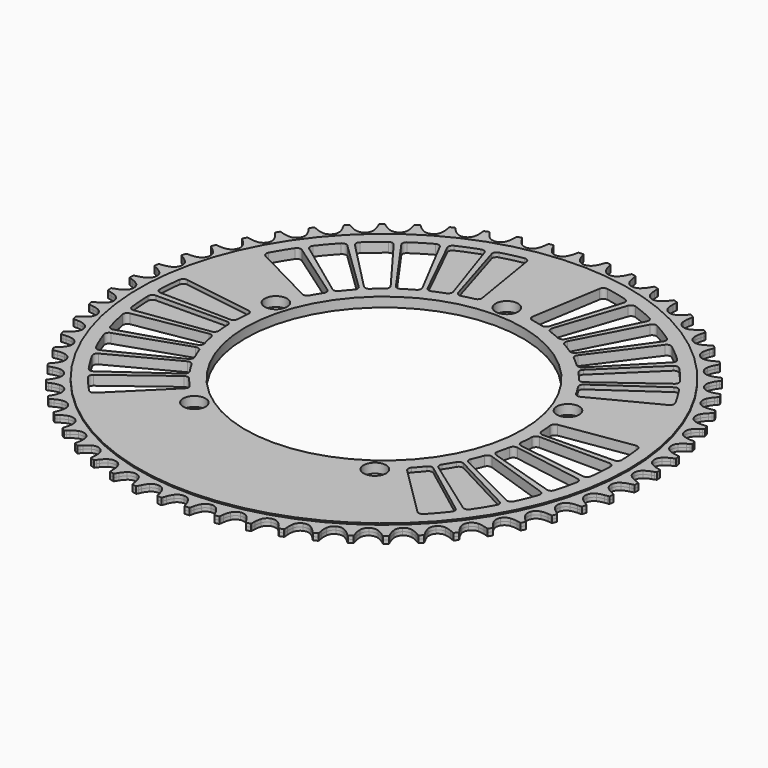
from build123d import *

# Parameters (mm, degrees)
F0_R     = 114.7609592
F0_R_2   = 5.25
F0_R_3   = 64.999997
F1_DEPTH = 2.25
F2_DEPTH = 1.58
F4_DEPTH = 4.5
F5_DEPTH = 2
F6_R     = 2


# Not quite as in the source:
# - the program builds the solid bodies; features that only make, move or delete a surface that nothing else refers to are left out


with BuildPart() as f1:
    # F0 (on Top) → F1 (new body, symmetric)
    with BuildSketch(Plane.XY):
        Circle(F0_R)
        with Locations((-42.3205431025, -58.2492303907)):
            Circle(F0_R_2, mode=Mode.SUBTRACT)
        with Locations((42.3205431025, -58.2492303907)):
            Circle(F0_R_2, mode=Mode.SUBTRACT)
        with Locations((-68.4760771621, 22.2492261907)):
            Circle(F0_R_2, mode=Mode.SUBTRACT)
        Circle(F0_R_3, mode=Mode.SUBTRACT)
        with Locations((68.4760771621, 22.2492261907)):
            Circle(F0_R_2, mode=Mode.SUBTRACT)
        with Locations((0, 72.0000084)):
            Circle(F0_R_2, mode=Mode.SUBTRACT)
    extrude(amount=F1_DEPTH, both=True)

    # F0 (on Top) → F2 (join, symmetric)
    with BuildSketch(Plane.XY):
        with BuildLine():
            ThreePointArc((0, 117.2608808999), (-1.8228579778, 117.698510644), (-3.2483562505, 118.9160021941))
            ThreePointArc((-3.2483562505, 118.9160021941), (-4.0685117692, 120.2255440434), (-4.6854512368, 121.6422093615))
            Line((-4.6854512368, 121.6422093615), (-5.0711986994, 122.7667517072))
            ThreePointArc((-5.0711986994, 122.7667517072), (-5.2354254241, 123.1948132929), (-5.4299253665, 123.6099962774))
            ThreePointArc((-5.4299253665, 123.6099962774), (-6.4754860684, 123.5596347897), (-7.5205832882, 123.5004295385))
            ThreePointArc((-7.5205832882, 123.5004295385), (-7.6706193003, 123.0671901897), (-7.789201754, 122.6243072031))
            Line((-7.789201754, 122.6243072031), (-8.0552893683, 121.4656036285))
            ThreePointArc((-8.0552893683, 121.4656036285), (-8.5207673283, 119.9922112167), (-9.1995455522, 118.6041135787))
            ThreePointArc((-9.1995455522, 118.6041135787), (-10.4899722755, 117.2442864308), (-12.2570996819, 116.6185135251))
            ThreePointArc((-12.2570996819, 116.6185135251), (-14.1157166175, 116.8632053445), (-15.6606683823, 117.9250222046))
            ThreePointArc((-15.6606683823, 117.9250222046), (-16.6132154005, 119.1416606507), (-17.3748570578, 120.4860775935))
            Line((-17.3748570578, 120.4860775935), (-17.8760380386, 121.5641379891))
            ThreePointArc((-17.8760380386, 121.5641379891), (-18.0841097318, 121.9726882415), (-18.3209426226, 122.36526603))
            ThreePointArc((-18.3209426226, 122.36526603), (-19.3555114246, 122.2058895744), (-20.3886948586, 122.0377662494))
            ThreePointArc((-20.3886948586, 122.0377662494), (-20.4926231144, 121.5912171974), (-20.564262083, 121.1383651284))
            Line((-20.564262083, 121.1383651284), (-20.7077745375, 119.9581953238))
            ThreePointArc((-20.7077745375, 119.9581953238), (-21.0166911159, 118.444218614), (-21.5466552087, 116.9927734754))
            ThreePointArc((-21.5466552087, 116.9927734754), (-22.6878721973, 115.5055092806), (-24.3799080147, 114.6984493121))
            ThreePointArc((-24.3799080147, 114.6984493121), (-26.2539205121, 114.7475223121), (-27.9013989542, 115.6420309946))
            ThreePointArc((-27.9013989542, 115.6420309946), (-28.9759011672, 116.7524362919), (-29.8739003088, 118.009875146))
            Line((-29.8739003088, 118.009875146), (-30.4850237643, 119.0296421363))
            ThreePointArc((-30.4850237643, 119.0296421363), (-30.7346607491, 119.4142048932), (-31.0112317974, 119.7798763215))
            ThreePointArc((-31.0112317974, 119.7798763215), (-32.0234737473, 119.5132310597), (-33.0334236215, 119.2380316553))
            ThreePointArc((-33.0334236215, 119.2380316553), (-33.0901054612, 118.7830653848), (-33.1140160532, 118.3252057755))
            Line((-33.1140160532, 118.3252057755), (-33.1333809954, 117.1364999283))
            ThreePointArc((-33.1333809954, 117.1364999283), (-33.2823516376, 115.5985263661), (-33.6576952018, 114.0996360636))
            ThreePointArc((-33.6576952018, 114.0996360636), (-34.6371990436, 112.5012295996), (-36.2356049734, 111.5217248863))
            ThreePointArc((-36.2356049734, 111.5217248863), (-38.1044809596, 111.3746414127), (-39.8364359603, 112.0920414932))
            ThreePointArc((-39.8364359603, 112.0920414932), (-41.0211208971, 113.0840478091), (-42.0456388566, 114.2407318113))
            Line((-42.0456388566, 114.2407318113), (-42.7600091902, 115.1910326156))
            ThreePointArc((-42.7600091902, 115.1910326156), (-43.0484763915, 115.5473945272), (-43.3617554271, 115.8821532224))
            ThreePointArc((-43.3617554271, 115.8821532224), (-44.3405801903, 115.5111605758), (-45.3162312826, 115.1319002342))
            ThreePointArc((-45.3162312826, 115.1319002342), (-45.3250456881, 114.6735014509), (-45.3009659341, 114.2156507071))
            Line((-45.3009659341, 114.2156507071), (-45.1959711976, 113.0314325272))
            ThreePointArc((-45.1959711976, 113.0314325272), (-45.18336375, 111.4863124728), (-45.399974443, 109.9563991622))
            ThreePointArc((-45.399974443, 109.9563991622), (-46.2070334888, 108.2643629048), (-47.6942970613, 107.1231451052))
            ThreePointArc((-47.6942970613, 107.1231451052), (-49.5375607399, 106.7815166354), (-51.3350166378, 107.3139481286))
            ThreePointArc((-51.3350166378, 107.3139481286), (-52.6169046423, 108.1766868341), (-53.7567165864, 109.2199431124))
            Line((-53.7567165864, 109.2199431124), (-54.5665070074, 110.0903660363))
            ThreePointArc((-54.5665070074, 110.0903660363), (-54.8906439181, 110.4146227268), (-55.2371985904, 110.7148010027))
            ThreePointArc((-55.2371985904, 110.7148010027), (-56.1718819578, 110.2435256444), (-57.1025448307, 109.7643596212))
            ThreePointArc((-57.1025448307, 109.7643596212), (-57.0633952296, 109.3075506382), (-56.9915889523, 108.8547250683))
            Line((-56.9915889523, 108.8547250683), (-56.7633848814, 107.6879690979))
            ThreePointArc((-56.7633848814, 107.6879690979), (-56.5893374739, 106.15263121), (-56.6448420636, 104.6084569418))
            ThreePointArc((-56.6448420636, 104.6084569418), (-57.2706140057, 102.8413291941), (-58.6304404499, 101.5509017294))
            ThreePointArc((-58.6304404499, 101.5509017294), (-60.4278966382, 101.0184712164), (-62.2711601305, 101.3601006913))
            ThreePointArc((-62.2711601305, 101.3601006913), (-63.6362065695, 102.0841194408), (-64.87882448, 103.0025178611))
            Line((-64.87882448, 103.0025178611), (-65.7751627549, 103.7835263689))
            ThreePointArc((-65.7751627549, 103.7835263689), (-66.1314180633, 104.0721252141), (-66.5074514467, 104.3344342547))
            ThreePointArc((-66.5074514467, 104.3344342547), (-67.3877528319, 103.768039576), (-68.2632309481, 103.1942177145))
            ThreePointArc((-68.2632309481, 103.1942177145), (-68.1765462717, 102.7440034266), (-68.0578001957, 102.3011642823))
            Line((-68.0578001957, 102.3011642823), (-67.708887042, 101.1646537441))
            ThreePointArc((-67.708887042, 101.1646537441), (-67.3753065744, 99.6559195058), (-67.2690969408, 98.1144025763))
            ThreePointArc((-67.2690969408, 98.1144025763), (-67.706725691, 96.2915443599), (-68.9242164638, 94.8660454234))
            ThreePointArc((-68.9242164638, 94.8660454234), (-70.6561718556, 94.1486462872), (-72.5250477616, 94.2957307799))
            ThreePointArc((-72.5250477616, 94.2957307799), (-73.9582969007, 94.8730970723), (-75.2901063959, 95.6565754694))
            Line((-75.2901063959, 95.6565754694), (-76.263172055, 96.3396126684))
            ThreePointArc((-76.263172055, 96.3396126684), (-76.6476425533, 96.5893917191), (-77.0490347475, 96.8109576116))
            ThreePointArc((-77.0490347475, 96.8109576116), (-77.8653093842, 96.1556491512), (-78.6760108223, 95.4934583638))
            ThreePointArc((-78.6760108223, 95.4934583638), (-78.5427408059, 95.0547714128), (-78.3783559381, 94.6267705326))
            Line((-78.3783559381, 94.6267705326), (-77.9125564672, 93.5329572738))
            ThreePointArc((-77.9125564672, 93.5329572738), (-77.4230977169, 92.0673566932), (-77.156337515, 90.5453862845))
            ThreePointArc((-77.156337515, 90.5453862845), (-77.401028321, 88.6867692154), (-78.4628443387, 87.1418168717))
            ThreePointArc((-78.4628443387, 87.1418168717), (-80.1103232685, 86.2473090875), (-81.9843357927, 86.1982371094))
            ThreePointArc((-81.9843357927, 86.1982371094), (-83.4700846543, 86.6226251989), (-84.8764941506, 87.2625996194))
            Line((-84.8764941506, 87.2625996194), (-85.915626083, 87.8401820112))
            ThreePointArc((-85.915626083, 87.8401820112), (-86.324099432, 88.0484046357), (-86.7464527, 88.2267998579))
            ThreePointArc((-86.7464527, 88.2267998579), (-87.4897573125, 87.4897573125), (-88.2267998579, 86.7464527))
            ThreePointArc((-88.2267998579, 86.7464527), (-88.0484046357, 86.324099432), (-87.8401820112, 85.915626083))
            Line((-87.8401820112, 85.915626083), (-87.2625996194, 84.8764941506))
            ThreePointArc((-87.2625996194, 84.8764941506), (-86.6226251989, 83.4700846543), (-86.1982371094, 81.9843357927))
            ThreePointArc((-86.1982371094, 81.9843357927), (-86.2473090875, 80.1103232685), (-87.1418168717, 78.4628443387))
            ThreePointArc((-87.1418168717, 78.4628443387), (-88.6867692154, 77.401028321), (-90.5453862845, 77.156337515))
            ThreePointArc((-90.5453862845, 77.156337515), (-92.0673566932, 77.4230977169), (-93.5329572738, 77.9125564672))
            Line((-93.5329572738, 77.9125564672), (-94.6267705326, 78.3783559381))
            ThreePointArc((-94.6267705326, 78.3783559381), (-95.0547714128, 78.5427408059), (-95.4934583638, 78.6760108223))
            ThreePointArc((-95.4934583638, 78.6760108223), (-96.1556491512, 77.8653093842), (-96.8109576116, 77.0490347475))
            ThreePointArc((-96.8109576116, 77.0490347475), (-96.5893917191, 76.6476425533), (-96.3396126684, 76.263172055))
            Line((-96.3396126684, 76.263172055), (-95.6565754694, 75.2901063959))
            ThreePointArc((-95.6565754694, 75.2901063959), (-94.8730970723, 73.9582969007), (-94.2957307799, 72.5250477616))
            ThreePointArc((-94.2957307799, 72.5250477616), (-94.1486462872, 70.6561718556), (-94.8660454234, 68.9242164638))
            ThreePointArc((-94.8660454234, 68.9242164638), (-96.2915443599, 67.706725691), (-98.1144025763, 67.2690969408))
            ThreePointArc((-98.1144025763, 67.2690969408), (-99.6559195058, 67.3753065744), (-101.1646537441, 67.708887042))
            Line((-101.1646537441, 67.708887042), (-102.3011642823, 68.0578001957))
            ThreePointArc((-102.3011642823, 68.0578001957), (-102.7440034266, 68.1765462717), (-103.1942177145, 68.2632309481))
            ThreePointArc((-103.1942177145, 68.2632309481), (-103.768039576, 67.3877528319), (-104.3344342547, 66.5074514467))
            ThreePointArc((-104.3344342547, 66.5074514467), (-104.0721252141, 66.1314180633), (-103.7835263689, 65.7751627549))
            Line((-103.7835263689, 65.7751627549), (-103.0025178611, 64.87882448))
            ThreePointArc((-103.0025178611, 64.87882448), (-102.0841194408, 63.6362065695), (-101.3601006913, 62.2711601305))
            ThreePointArc((-101.3601006913, 62.2711601305), (-101.0184712164, 60.4278966382), (-101.5509017294, 58.6304404499))
            ThreePointArc((-101.5509017294, 58.6304404499), (-102.8413291941, 57.2706140057), (-104.6084569418, 56.6448420636))
            ThreePointArc((-104.6084569418, 56.6448420636), (-106.15263121, 56.5893374739), (-107.6879690979, 56.7633848814))
            Line((-107.6879690979, 56.7633848814), (-108.8547250683, 56.9915889523))
            ThreePointArc((-108.8547250683, 56.9915889523), (-109.3075506382, 57.0633952296), (-109.7643596212, 57.1025448307))
            ThreePointArc((-109.7643596212, 57.1025448307), (-110.2435256444, 56.1718819578), (-110.7148010027, 55.2371985904))
            ThreePointArc((-110.7148010027, 55.2371985904), (-110.4146227268, 54.8906439181), (-110.0903660363, 54.5665070074))
            Line((-110.0903660363, 54.5665070074), (-109.2199431124, 53.7567165864))
            ThreePointArc((-109.2199431124, 53.7567165864), (-108.1766868341, 52.6169046423), (-107.3139481286, 51.3350166378))
            ThreePointArc((-107.3139481286, 51.3350166378), (-106.7815166354, 49.5375607399), (-107.1231451052, 47.6942970613))
            ThreePointArc((-107.1231451052, 47.6942970613), (-108.2643629048, 46.2070334888), (-109.9563991622, 45.399974443))
            ThreePointArc((-109.9563991622, 45.399974443), (-111.4863124728, 45.18336375), (-113.0314325272, 45.1959711976))
            Line((-113.0314325272, 45.1959711976), (-114.2156507071, 45.3009659341))
            ThreePointArc((-114.2156507071, 45.3009659341), (-114.6735014509, 45.3250456881), (-115.1319002342, 45.3162312826))
            ThreePointArc((-115.1319002342, 45.3162312826), (-115.5111605758, 44.3405801903), (-115.8821532224, 43.3617554271))
            ThreePointArc((-115.8821532224, 43.3617554271), (-115.5473945272, 43.0484763915), (-115.1910326156, 42.7600091902))
            Line((-115.1910326156, 42.7600091902), (-114.2407318113, 42.0456388566))
            ThreePointArc((-114.2407318113, 42.0456388566), (-113.0840478091, 41.0211208971), (-112.0920414932, 39.8364359603))
            ThreePointArc((-112.0920414932, 39.8364359603), (-111.3746414127, 38.1044809596), (-111.5217248863, 36.2356049734))
            ThreePointArc((-111.5217248863, 36.2356049734), (-112.5012295996, 34.6371990436), (-114.0996360636, 33.6576952018))
            ThreePointArc((-114.0996360636, 33.6576952018), (-115.5985263661, 33.2823516376), (-117.1364999283, 33.1333809954))
            Line((-117.1364999283, 33.1333809954), (-118.3252057755, 33.1140160532))
            ThreePointArc((-118.3252057755, 33.1140160532), (-118.7830653848, 33.0901054612), (-119.2380316553, 33.0334236215))
            ThreePointArc((-119.2380316553, 33.0334236215), (-119.5132310597, 32.0234737473), (-119.7798763215, 31.0112317974))
            ThreePointArc((-119.7798763215, 31.0112317974), (-119.4142048932, 30.7346607491), (-119.0296421363, 30.4850237643))
            Line((-119.0296421363, 30.4850237643), (-118.009875146, 29.8739003088))
            ThreePointArc((-118.009875146, 29.8739003088), (-116.7524362919, 28.9759011672), (-115.6420309946, 27.9013989542))
            ThreePointArc((-115.6420309946, 27.9013989542), (-114.7475223121, 26.2539205121), (-114.6984493121, 24.3799080147))
            ThreePointArc((-114.6984493121, 24.3799080147), (-115.5055092806, 22.6878721973), (-116.9927734754, 21.5466552087))
            ThreePointArc((-116.9927734754, 21.5466552087), (-118.444218614, 21.0166911159), (-119.9581953238, 20.7077745375))
            Line((-119.9581953238, 20.7077745375), (-121.1383651284, 20.564262083))
            ThreePointArc((-121.1383651284, 20.564262083), (-121.5912171974, 20.4926231144), (-122.0377662494, 20.3886948586))
            ThreePointArc((-122.0377662494, 20.3886948586), (-122.2058895744, 19.3555114246), (-122.36526603, 18.3209426226))
            ThreePointArc((-122.36526603, 18.3209426226), (-121.9726882415, 18.0841097318), (-121.5641379891, 17.8760380386))
            Line((-121.5641379891, 17.8760380386), (-120.4860775935, 17.3748570578))
            ThreePointArc((-120.4860775935, 17.3748570578), (-119.1416606507, 16.6132154005), (-117.9250222046, 15.6606683823))
            ThreePointArc((-117.9250222046, 15.6606683823), (-116.8632053445, 14.1157166175), (-116.6185135251, 12.2570996819))
            ThreePointArc((-116.6185135251, 12.2570996819), (-117.2442864308, 10.4899722755), (-118.6041135787, 9.1995455522))
            ThreePointArc((-118.6041135787, 9.1995455522), (-119.9922112167, 8.5207673283), (-121.4656036285, 8.0552893683))
            Line((-121.4656036285, 8.0552893683), (-122.6243072031, 7.789201754))
            ThreePointArc((-122.6243072031, 7.789201754), (-123.0671901897, 7.6706193003), (-123.5004295385, 7.5205832882))
            ThreePointArc((-123.5004295385, 7.5205832882), (-123.5596347897, 6.4754860684), (-123.6099962774, 5.4299253665))
            ThreePointArc((-123.6099962774, 5.4299253665), (-123.1948132929, 5.2354254241), (-122.7667517072, 5.0711986994))
            Line((-122.7667517072, 5.0711986994), (-121.6422093615, 4.6854512368))
            ThreePointArc((-121.6422093615, 4.6854512368), (-120.2255440434, 4.0685117692), (-118.9160021941, 3.2483562505))
            ThreePointArc((-118.9160021941, 3.2483562505), (-117.698510644, 1.8228579778), (-117.2608808999, 0))
            ThreePointArc((-117.2608808999, 0), (-117.698510644, -1.8228579778), (-118.9160021941, -3.2483562505))
            ThreePointArc((-118.9160021941, -3.2483562505), (-120.2255440434, -4.0685117692), (-121.6422093615, -4.6854512368))
            Line((-121.6422093615, -4.6854512368), (-122.7667517072, -5.0711986994))
            ThreePointArc((-122.7667517072, -5.0711986994), (-123.1948132929, -5.2354254241), (-123.6099962774, -5.4299253665))
            ThreePointArc((-123.6099962774, -5.4299253665), (-123.5596347897, -6.4754860684), (-123.5004295385, -7.5205832882))
            ThreePointArc((-123.5004295385, -7.5205832882), (-123.0671901897, -7.6706193003), (-122.6243072031, -7.789201754))
            Line((-122.6243072031, -7.789201754), (-121.4656036285, -8.0552893683))
            ThreePointArc((-121.4656036285, -8.0552893683), (-119.9922112167, -8.5207673283), (-118.6041135787, -9.1995455522))
            ThreePointArc((-118.6041135787, -9.1995455522), (-117.2442864308, -10.4899722755), (-116.6185135251, -12.2570996819))
            ThreePointArc((-116.6185135251, -12.2570996819), (-116.8632053445, -14.1157166175), (-117.9250222046, -15.6606683823))
            ThreePointArc((-117.9250222046, -15.6606683823), (-119.1416606507, -16.6132154005), (-120.4860775935, -17.3748570578))
            Line((-120.4860775935, -17.3748570578), (-121.5641379891, -17.8760380386))
            ThreePointArc((-121.5641379891, -17.8760380386), (-121.9726882415, -18.0841097318), (-122.36526603, -18.3209426226))
            ThreePointArc((-122.36526603, -18.3209426226), (-122.2058895744, -19.3555114246), (-122.0377662494, -20.3886948586))
            ThreePointArc((-122.0377662494, -20.3886948586), (-121.5912171974, -20.4926231144), (-121.1383651284, -20.564262083))
            Line((-121.1383651284, -20.564262083), (-119.9581953238, -20.7077745375))
            ThreePointArc((-119.9581953238, -20.7077745375), (-118.444218614, -21.0166911159), (-116.9927734754, -21.5466552087))
            ThreePointArc((-116.9927734754, -21.5466552087), (-115.5055092806, -22.6878721973), (-114.6984493121, -24.3799080147))
            ThreePointArc((-114.6984493121, -24.3799080147), (-114.7475223121, -26.2539205121), (-115.6420309946, -27.9013989542))
            ThreePointArc((-115.6420309946, -27.9013989542), (-116.7524362919, -28.9759011672), (-118.009875146, -29.8739003088))
            Line((-118.009875146, -29.8739003088), (-119.0296421363, -30.4850237643))
            ThreePointArc((-119.0296421363, -30.4850237643), (-119.4142048932, -30.7346607491), (-119.7798763215, -31.0112317974))
            ThreePointArc((-119.7798763215, -31.0112317974), (-119.5132310597, -32.0234737473), (-119.2380316553, -33.0334236215))
            ThreePointArc((-119.2380316553, -33.0334236215), (-118.7830653848, -33.0901054612), (-118.3252057755, -33.1140160532))
            Line((-118.3252057755, -33.1140160532), (-117.1364999283, -33.1333809954))
            ThreePointArc((-117.1364999283, -33.1333809954), (-115.5985263661, -33.2823516376), (-114.0996360636, -33.6576952018))
            ThreePointArc((-114.0996360636, -33.6576952018), (-112.5012295996, -34.6371990436), (-111.5217248863, -36.2356049734))
            ThreePointArc((-111.5217248863, -36.2356049734), (-111.3746414127, -38.1044809596), (-112.0920414932, -39.8364359603))
            ThreePointArc((-112.0920414932, -39.8364359603), (-113.0840478091, -41.0211208971), (-114.2407318113, -42.0456388566))
            Line((-114.2407318113, -42.0456388566), (-115.1910326156, -42.7600091902))
            ThreePointArc((-115.1910326156, -42.7600091902), (-115.5473945272, -43.0484763915), (-115.8821532224, -43.3617554271))
            ThreePointArc((-115.8821532224, -43.3617554271), (-115.5111605758, -44.3405801903), (-115.1319002342, -45.3162312826))
            ThreePointArc((-115.1319002342, -45.3162312826), (-114.6735014509, -45.3250456881), (-114.2156507071, -45.3009659341))
            Line((-114.2156507071, -45.3009659341), (-113.0314325272, -45.1959711976))
            ThreePointArc((-113.0314325272, -45.1959711976), (-111.4863124728, -45.18336375), (-109.9563991622, -45.399974443))
            ThreePointArc((-109.9563991622, -45.399974443), (-108.2643629048, -46.2070334888), (-107.1231451052, -47.6942970613))
            ThreePointArc((-107.1231451052, -47.6942970613), (-106.7815166354, -49.5375607399), (-107.3139481286, -51.3350166378))
            ThreePointArc((-107.3139481286, -51.3350166378), (-108.1766868341, -52.6169046423), (-109.2199431124, -53.7567165864))
            Line((-109.2199431124, -53.7567165864), (-110.0903660363, -54.5665070074))
            ThreePointArc((-110.0903660363, -54.5665070074), (-110.4146227268, -54.8906439181), (-110.7148010027, -55.2371985904))
            ThreePointArc((-110.7148010027, -55.2371985904), (-110.2435256444, -56.1718819578), (-109.7643596212, -57.1025448307))
            ThreePointArc((-109.7643596212, -57.1025448307), (-109.3075506382, -57.0633952296), (-108.8547250683, -56.9915889523))
            Line((-108.8547250683, -56.9915889523), (-107.6879690979, -56.7633848814))
            ThreePointArc((-107.6879690979, -56.7633848814), (-106.15263121, -56.5893374739), (-104.6084569418, -56.6448420636))
            ThreePointArc((-104.6084569418, -56.6448420636), (-102.8413291941, -57.2706140057), (-101.5509017294, -58.6304404499))
            ThreePointArc((-101.5509017294, -58.6304404499), (-101.0184712164, -60.4278966382), (-101.3601006913, -62.2711601305))
            ThreePointArc((-101.3601006913, -62.2711601305), (-102.0841194408, -63.6362065695), (-103.0025178611, -64.87882448))
            Line((-103.0025178611, -64.87882448), (-103.7835263689, -65.7751627549))
            ThreePointArc((-103.7835263689, -65.7751627549), (-104.0721252141, -66.1314180633), (-104.3344342547, -66.5074514467))
            ThreePointArc((-104.3344342547, -66.5074514467), (-103.768039576, -67.3877528319), (-103.1942177145, -68.2632309481))
            ThreePointArc((-103.1942177145, -68.2632309481), (-102.7440034266, -68.1765462717), (-102.3011642823, -68.0578001957))
            Line((-102.3011642823, -68.0578001957), (-101.1646537441, -67.708887042))
            ThreePointArc((-101.1646537441, -67.708887042), (-99.6559195058, -67.3753065744), (-98.1144025763, -67.2690969408))
            ThreePointArc((-98.1144025763, -67.2690969408), (-96.2915443599, -67.706725691), (-94.8660454234, -68.9242164638))
            ThreePointArc((-94.8660454234, -68.9242164638), (-94.1486462872, -70.6561718556), (-94.2957307799, -72.5250477616))
            ThreePointArc((-94.2957307799, -72.5250477616), (-94.8730970723, -73.9582969007), (-95.6565754694, -75.2901063959))
            Line((-95.6565754694, -75.2901063959), (-96.3396126684, -76.263172055))
            ThreePointArc((-96.3396126684, -76.263172055), (-96.5893917191, -76.6476425533), (-96.8109576116, -77.0490347475))
            ThreePointArc((-96.8109576116, -77.0490347475), (-96.1556491512, -77.8653093842), (-95.4934583638, -78.6760108223))
            ThreePointArc((-95.4934583638, -78.6760108223), (-95.0547714128, -78.5427408059), (-94.6267705326, -78.3783559381))
            Line((-94.6267705326, -78.3783559381), (-93.5329572738, -77.9125564672))
            ThreePointArc((-93.5329572738, -77.9125564672), (-92.0673566932, -77.4230977169), (-90.5453862845, -77.156337515))
            ThreePointArc((-90.5453862845, -77.156337515), (-88.6867692154, -77.401028321), (-87.1418168717, -78.4628443387))
            ThreePointArc((-87.1418168717, -78.4628443387), (-86.2473090875, -80.1103232685), (-86.1982371094, -81.9843357927))
            ThreePointArc((-86.1982371094, -81.9843357927), (-86.6226251989, -83.4700846543), (-87.2625996194, -84.8764941506))
            Line((-87.2625996194, -84.8764941506), (-87.8401820112, -85.915626083))
            ThreePointArc((-87.8401820112, -85.915626083), (-88.0484046357, -86.324099432), (-88.2267998579, -86.7464527))
            ThreePointArc((-88.2267998579, -86.7464527), (-87.4897573125, -87.4897573125), (-86.7464527, -88.2267998579))
            ThreePointArc((-86.7464527, -88.2267998579), (-86.324099432, -88.0484046357), (-85.915626083, -87.8401820112))
            Line((-85.915626083, -87.8401820112), (-84.8764941506, -87.2625996194))
            ThreePointArc((-84.8764941506, -87.2625996194), (-83.4700846543, -86.6226251989), (-81.9843357927, -86.1982371094))
            ThreePointArc((-81.9843357927, -86.1982371094), (-80.1103232685, -86.2473090875), (-78.4628443387, -87.1418168717))
            ThreePointArc((-78.4628443387, -87.1418168717), (-77.401028321, -88.6867692154), (-77.156337515, -90.5453862845))
            ThreePointArc((-77.156337515, -90.5453862845), (-77.4230977169, -92.0673566932), (-77.9125564672, -93.5329572738))
            Line((-77.9125564672, -93.5329572738), (-78.3783559381, -94.6267705326))
            ThreePointArc((-78.3783559381, -94.6267705326), (-78.5427408059, -95.0547714128), (-78.6760108223, -95.4934583638))
            ThreePointArc((-78.6760108223, -95.4934583638), (-77.8653093842, -96.1556491512), (-77.0490347475, -96.8109576116))
            ThreePointArc((-77.0490347475, -96.8109576116), (-76.6476425533, -96.5893917191), (-76.263172055, -96.3396126684))
            Line((-76.263172055, -96.3396126684), (-75.2901063959, -95.6565754694))
            ThreePointArc((-75.2901063959, -95.6565754694), (-73.9582969007, -94.8730970723), (-72.5250477616, -94.2957307799))
            ThreePointArc((-72.5250477616, -94.2957307799), (-70.6561718556, -94.1486462872), (-68.9242164638, -94.8660454234))
            ThreePointArc((-68.9242164638, -94.8660454234), (-67.706725691, -96.2915443599), (-67.2690969408, -98.1144025763))
            ThreePointArc((-67.2690969408, -98.1144025763), (-67.3753065744, -99.6559195058), (-67.708887042, -101.1646537441))
            Line((-67.708887042, -101.1646537441), (-68.0578001957, -102.3011642823))
            ThreePointArc((-68.0578001957, -102.3011642823), (-68.1765462717, -102.7440034266), (-68.2632309481, -103.1942177145))
            ThreePointArc((-68.2632309481, -103.1942177145), (-67.3877528319, -103.768039576), (-66.5074514467, -104.3344342547))
            ThreePointArc((-66.5074514467, -104.3344342547), (-66.1314180633, -104.0721252141), (-65.7751627549, -103.7835263689))
            Line((-65.7751627549, -103.7835263689), (-64.87882448, -103.0025178611))
            ThreePointArc((-64.87882448, -103.0025178611), (-63.6362065695, -102.0841194408), (-62.2711601305, -101.3601006913))
            ThreePointArc((-62.2711601305, -101.3601006913), (-60.4278966382, -101.0184712164), (-58.6304404499, -101.5509017294))
            ThreePointArc((-58.6304404499, -101.5509017294), (-57.2706140057, -102.8413291941), (-56.6448420636, -104.6084569418))
            ThreePointArc((-56.6448420636, -104.6084569418), (-56.5893374739, -106.15263121), (-56.7633848814, -107.6879690979))
            Line((-56.7633848814, -107.6879690979), (-56.9915889523, -108.8547250683))
            ThreePointArc((-56.9915889523, -108.8547250683), (-57.0633952296, -109.3075506382), (-57.1025448307, -109.7643596212))
            ThreePointArc((-57.1025448307, -109.7643596212), (-56.1718819578, -110.2435256444), (-55.2371985904, -110.7148010027))
            ThreePointArc((-55.2371985904, -110.7148010027), (-54.8906439181, -110.4146227268), (-54.5665070074, -110.0903660363))
            Line((-54.5665070074, -110.0903660363), (-53.7567165864, -109.2199431124))
            ThreePointArc((-53.7567165864, -109.2199431124), (-52.6169046423, -108.1766868341), (-51.3350166378, -107.3139481286))
            ThreePointArc((-51.3350166378, -107.3139481286), (-49.5375607399, -106.7815166354), (-47.6942970613, -107.1231451052))
            ThreePointArc((-47.6942970613, -107.1231451052), (-46.2070334888, -108.2643629048), (-45.399974443, -109.9563991622))
            ThreePointArc((-45.399974443, -109.9563991622), (-45.18336375, -111.4863124728), (-45.1959711976, -113.0314325272))
            Line((-45.1959711976, -113.0314325272), (-45.3009659341, -114.2156507071))
            ThreePointArc((-45.3009659341, -114.2156507071), (-45.3250456881, -114.6735014509), (-45.3162312826, -115.1319002342))
            ThreePointArc((-45.3162312826, -115.1319002342), (-44.3405801903, -115.5111605758), (-43.3617554271, -115.8821532224))
            ThreePointArc((-43.3617554271, -115.8821532224), (-43.0484763915, -115.5473945272), (-42.7600091902, -115.1910326156))
            Line((-42.7600091902, -115.1910326156), (-42.0456388566, -114.2407318113))
            ThreePointArc((-42.0456388566, -114.2407318113), (-41.0211208971, -113.0840478091), (-39.8364359603, -112.0920414932))
            ThreePointArc((-39.8364359603, -112.0920414932), (-38.1044809596, -111.3746414127), (-36.2356049734, -111.5217248863))
            ThreePointArc((-36.2356049734, -111.5217248863), (-34.6371990436, -112.5012295996), (-33.6576952018, -114.0996360636))
            ThreePointArc((-33.6576952018, -114.0996360636), (-33.2823516376, -115.5985263661), (-33.1333809954, -117.1364999283))
            Line((-33.1333809954, -117.1364999283), (-33.1140160532, -118.3252057755))
            ThreePointArc((-33.1140160532, -118.3252057755), (-33.0901054612, -118.7830653848), (-33.0334236215, -119.2380316553))
            ThreePointArc((-33.0334236215, -119.2380316553), (-32.0234737473, -119.5132310597), (-31.0112317974, -119.7798763215))
            ThreePointArc((-31.0112317974, -119.7798763215), (-30.7346607491, -119.4142048932), (-30.4850237643, -119.0296421363))
            Line((-30.4850237643, -119.0296421363), (-29.8739003088, -118.009875146))
            ThreePointArc((-29.8739003088, -118.009875146), (-28.9759011672, -116.7524362919), (-27.9013989542, -115.6420309946))
            ThreePointArc((-27.9013989542, -115.6420309946), (-26.2539205121, -114.7475223121), (-24.3799080147, -114.6984493121))
            ThreePointArc((-24.3799080147, -114.6984493121), (-22.6878721973, -115.5055092806), (-21.5466552087, -116.9927734754))
            ThreePointArc((-21.5466552087, -116.9927734754), (-21.0166911159, -118.444218614), (-20.7077745375, -119.9581953238))
            Line((-20.7077745375, -119.9581953238), (-20.564262083, -121.1383651284))
            ThreePointArc((-20.564262083, -121.1383651284), (-20.4926231144, -121.5912171974), (-20.3886948586, -122.0377662494))
            ThreePointArc((-20.3886948586, -122.0377662494), (-19.3555114246, -122.2058895744), (-18.3209426226, -122.36526603))
            ThreePointArc((-18.3209426226, -122.36526603), (-18.0841097318, -121.9726882415), (-17.8760380386, -121.5641379891))
            Line((-17.8760380386, -121.5641379891), (-17.3748570578, -120.4860775935))
            ThreePointArc((-17.3748570578, -120.4860775935), (-16.6132154005, -119.1416606507), (-15.6606683823, -117.9250222046))
            ThreePointArc((-15.6606683823, -117.9250222046), (-14.1157166175, -116.8632053445), (-12.2570996819, -116.6185135251))
            ThreePointArc((-12.2570996819, -116.6185135251), (-10.4899722755, -117.2442864308), (-9.1995455522, -118.6041135787))
            ThreePointArc((-9.1995455522, -118.6041135787), (-8.5207673283, -119.9922112167), (-8.0552893683, -121.4656036285))
            Line((-8.0552893683, -121.4656036285), (-7.789201754, -122.6243072031))
            ThreePointArc((-7.789201754, -122.6243072031), (-7.6706193003, -123.0671901897), (-7.5205832882, -123.5004295385))
            ThreePointArc((-7.5205832882, -123.5004295385), (-6.4754860684, -123.5596347897), (-5.4299253665, -123.6099962774))
            ThreePointArc((-5.4299253665, -123.6099962774), (-5.2354254241, -123.1948132929), (-5.0711986994, -122.7667517072))
            Line((-5.0711986994, -122.7667517072), (-4.6854512368, -121.6422093615))
            ThreePointArc((-4.6854512368, -121.6422093615), (-4.0685117692, -120.2255440434), (-3.2483562505, -118.9160021941))
            ThreePointArc((-3.2483562505, -118.9160021941), (-1.8228579778, -117.698510644), (0, -117.2608808999))
            ThreePointArc((0, -117.2608808999), (1.8228579778, -117.698510644), (3.2483562505, -118.9160021941))
            ThreePointArc((3.2483562505, -118.9160021941), (4.0685117692, -120.2255440434), (4.6854512368, -121.6422093615))
            Line((4.6854512368, -121.6422093615), (5.0711986994, -122.7667517072))
            ThreePointArc((5.0711986994, -122.7667517072), (5.2354254241, -123.1948132929), (5.4299253665, -123.6099962774))
            ThreePointArc((5.4299253665, -123.6099962774), (6.4754860684, -123.5596347897), (7.5205832882, -123.5004295385))
            ThreePointArc((7.5205832882, -123.5004295385), (7.6706193003, -123.0671901897), (7.789201754, -122.6243072031))
            Line((7.789201754, -122.6243072031), (8.0552893683, -121.4656036285))
            ThreePointArc((8.0552893683, -121.4656036285), (8.5207673283, -119.9922112167), (9.1995455522, -118.6041135787))
            ThreePointArc((9.1995455522, -118.6041135787), (10.4899722755, -117.2442864308), (12.2570996819, -116.6185135251))
            ThreePointArc((12.2570996819, -116.6185135251), (14.1157166175, -116.8632053445), (15.6606683823, -117.9250222046))
            ThreePointArc((15.6606683823, -117.9250222046), (16.6132154005, -119.1416606507), (17.3748570578, -120.4860775935))
            Line((17.3748570578, -120.4860775935), (17.8760380386, -121.5641379891))
            ThreePointArc((17.8760380386, -121.5641379891), (18.0841097318, -121.9726882415), (18.3209426226, -122.36526603))
            ThreePointArc((18.3209426226, -122.36526603), (19.3555114246, -122.2058895744), (20.3886948586, -122.0377662494))
            ThreePointArc((20.3886948586, -122.0377662494), (20.4926231144, -121.5912171974), (20.564262083, -121.1383651284))
            Line((20.564262083, -121.1383651284), (20.7077745375, -119.9581953238))
            ThreePointArc((20.7077745375, -119.9581953238), (21.0166911159, -118.444218614), (21.5466552087, -116.9927734754))
            ThreePointArc((21.5466552087, -116.9927734754), (22.6878721973, -115.5055092806), (24.3799080147, -114.6984493121))
            ThreePointArc((24.3799080147, -114.6984493121), (26.2539205121, -114.7475223121), (27.9013989542, -115.6420309946))
            ThreePointArc((27.9013989542, -115.6420309946), (28.9759011672, -116.7524362919), (29.8739003088, -118.009875146))
            Line((29.8739003088, -118.009875146), (30.4850237643, -119.0296421363))
            ThreePointArc((30.4850237643, -119.0296421363), (30.7346607491, -119.4142048932), (31.0112317974, -119.7798763215))
            ThreePointArc((31.0112317974, -119.7798763215), (32.0234737473, -119.5132310597), (33.0334236215, -119.2380316553))
            ThreePointArc((33.0334236215, -119.2380316553), (33.0901054612, -118.7830653848), (33.1140160532, -118.3252057755))
            Line((33.1140160532, -118.3252057755), (33.1333809954, -117.1364999283))
            ThreePointArc((33.1333809954, -117.1364999283), (33.2823516376, -115.5985263661), (33.6576952018, -114.0996360636))
            ThreePointArc((33.6576952018, -114.0996360636), (34.6371990436, -112.5012295996), (36.2356049734, -111.5217248863))
            ThreePointArc((36.2356049734, -111.5217248863), (38.1044809596, -111.3746414127), (39.8364359603, -112.0920414932))
            ThreePointArc((39.8364359603, -112.0920414932), (41.0211208971, -113.0840478091), (42.0456388566, -114.2407318113))
            Line((42.0456388566, -114.2407318113), (42.7600091902, -115.1910326156))
            ThreePointArc((42.7600091902, -115.1910326156), (43.0484763915, -115.5473945272), (43.3617554271, -115.8821532224))
            ThreePointArc((43.3617554271, -115.8821532224), (44.3405801903, -115.5111605758), (45.3162312826, -115.1319002342))
            ThreePointArc((45.3162312826, -115.1319002342), (45.3250456881, -114.6735014509), (45.3009659341, -114.2156507071))
            Line((45.3009659341, -114.2156507071), (45.1959711976, -113.0314325272))
            ThreePointArc((45.1959711976, -113.0314325272), (45.18336375, -111.4863124728), (45.399974443, -109.9563991622))
            ThreePointArc((45.399974443, -109.9563991622), (46.2070334888, -108.2643629048), (47.6942970613, -107.1231451052))
            ThreePointArc((47.6942970613, -107.1231451052), (49.5375607399, -106.7815166354), (51.3350166378, -107.3139481286))
            ThreePointArc((51.3350166378, -107.3139481286), (52.6169046423, -108.1766868341), (53.7567165864, -109.2199431124))
            Line((53.7567165864, -109.2199431124), (54.5665070074, -110.0903660363))
            ThreePointArc((54.5665070074, -110.0903660363), (54.8906439181, -110.4146227268), (55.2371985904, -110.7148010027))
            ThreePointArc((55.2371985904, -110.7148010027), (56.1718819578, -110.2435256444), (57.1025448307, -109.7643596212))
            ThreePointArc((57.1025448307, -109.7643596212), (57.0633952296, -109.3075506382), (56.9915889523, -108.8547250683))
            Line((56.9915889523, -108.8547250683), (56.7633848814, -107.6879690979))
            ThreePointArc((56.7633848814, -107.6879690979), (56.5893374739, -106.15263121), (56.6448420636, -104.6084569418))
            ThreePointArc((56.6448420636, -104.6084569418), (57.2706140057, -102.8413291941), (58.6304404499, -101.5509017294))
            ThreePointArc((58.6304404499, -101.5509017294), (60.4278966382, -101.0184712164), (62.2711601305, -101.3601006913))
            ThreePointArc((62.2711601305, -101.3601006913), (63.6362065695, -102.0841194408), (64.87882448, -103.0025178611))
            Line((64.87882448, -103.0025178611), (65.7751627549, -103.7835263689))
            ThreePointArc((65.7751627549, -103.7835263689), (66.1314180633, -104.0721252141), (66.5074514467, -104.3344342547))
            ThreePointArc((66.5074514467, -104.3344342547), (67.3877528319, -103.768039576), (68.2632309481, -103.1942177145))
            ThreePointArc((68.2632309481, -103.1942177145), (68.1765462717, -102.7440034266), (68.0578001957, -102.3011642823))
            Line((68.0578001957, -102.3011642823), (67.708887042, -101.1646537441))
            ThreePointArc((67.708887042, -101.1646537441), (67.3753065744, -99.6559195058), (67.2690969408, -98.1144025763))
            ThreePointArc((67.2690969408, -98.1144025763), (67.706725691, -96.2915443599), (68.9242164638, -94.8660454234))
            ThreePointArc((68.9242164638, -94.8660454234), (70.6561718556, -94.1486462872), (72.5250477616, -94.2957307799))
            ThreePointArc((72.5250477616, -94.2957307799), (73.9582969007, -94.8730970723), (75.2901063959, -95.6565754694))
            Line((75.2901063959, -95.6565754694), (76.263172055, -96.3396126684))
            ThreePointArc((76.263172055, -96.3396126684), (76.6476425533, -96.5893917191), (77.0490347475, -96.8109576116))
            ThreePointArc((77.0490347475, -96.8109576116), (77.8653093842, -96.1556491512), (78.6760108223, -95.4934583638))
            ThreePointArc((78.6760108223, -95.4934583638), (78.5427408059, -95.0547714128), (78.3783559381, -94.6267705326))
            Line((78.3783559381, -94.6267705326), (77.9125564672, -93.5329572738))
            ThreePointArc((77.9125564672, -93.5329572738), (77.4230977169, -92.0673566932), (77.156337515, -90.5453862845))
            ThreePointArc((77.156337515, -90.5453862845), (77.401028321, -88.6867692154), (78.4628443387, -87.1418168717))
            ThreePointArc((78.4628443387, -87.1418168717), (80.1103232685, -86.2473090875), (81.9843357927, -86.1982371094))
            ThreePointArc((81.9843357927, -86.1982371094), (83.4700846543, -86.6226251989), (84.8764941506, -87.2625996194))
            Line((84.8764941506, -87.2625996194), (85.915626083, -87.8401820112))
            ThreePointArc((85.915626083, -87.8401820112), (86.324099432, -88.0484046357), (86.7464527, -88.2267998579))
            ThreePointArc((86.7464527, -88.2267998579), (87.4897573125, -87.4897573125), (88.2267998579, -86.7464527))
            ThreePointArc((88.2267998579, -86.7464527), (88.0484046357, -86.324099432), (87.8401820112, -85.915626083))
            Line((87.8401820112, -85.915626083), (87.2625996194, -84.8764941506))
            ThreePointArc((87.2625996194, -84.8764941506), (86.6226251989, -83.4700846543), (86.1982371094, -81.9843357927))
            ThreePointArc((86.1982371094, -81.9843357927), (86.2473090875, -80.1103232685), (87.1418168717, -78.4628443387))
            ThreePointArc((87.1418168717, -78.4628443387), (88.6867692154, -77.401028321), (90.5453862845, -77.156337515))
            ThreePointArc((90.5453862845, -77.156337515), (92.0673566932, -77.4230977169), (93.5329572738, -77.9125564672))
            Line((93.5329572738, -77.9125564672), (94.6267705326, -78.3783559381))
            ThreePointArc((94.6267705326, -78.3783559381), (95.0547714128, -78.5427408059), (95.4934583638, -78.6760108223))
            ThreePointArc((95.4934583638, -78.6760108223), (96.1556491512, -77.8653093842), (96.8109576116, -77.0490347475))
            ThreePointArc((96.8109576116, -77.0490347475), (96.5893917191, -76.6476425533), (96.3396126684, -76.263172055))
            Line((96.3396126684, -76.263172055), (95.6565754694, -75.2901063959))
            ThreePointArc((95.6565754694, -75.2901063959), (94.8730970723, -73.9582969007), (94.2957307799, -72.5250477616))
            ThreePointArc((94.2957307799, -72.5250477616), (94.1486462872, -70.6561718556), (94.8660454234, -68.9242164638))
            ThreePointArc((94.8660454234, -68.9242164638), (96.2915443599, -67.706725691), (98.1144025763, -67.2690969408))
            ThreePointArc((98.1144025763, -67.2690969408), (99.6559195058, -67.3753065744), (101.1646537441, -67.708887042))
            Line((101.1646537441, -67.708887042), (102.3011642823, -68.0578001957))
            ThreePointArc((102.3011642823, -68.0578001957), (102.7440034266, -68.1765462717), (103.1942177145, -68.2632309481))
            ThreePointArc((103.1942177145, -68.2632309481), (103.768039576, -67.3877528319), (104.3344342547, -66.5074514467))
            ThreePointArc((104.3344342547, -66.5074514467), (104.0721252141, -66.1314180633), (103.7835263689, -65.7751627549))
            Line((103.7835263689, -65.7751627549), (103.0025178611, -64.87882448))
            ThreePointArc((103.0025178611, -64.87882448), (102.0841194408, -63.6362065695), (101.3601006913, -62.2711601305))
            ThreePointArc((101.3601006913, -62.2711601305), (101.0184712164, -60.4278966382), (101.5509017294, -58.6304404499))
            ThreePointArc((101.5509017294, -58.6304404499), (102.8413291941, -57.2706140057), (104.6084569418, -56.6448420636))
            ThreePointArc((104.6084569418, -56.6448420636), (106.15263121, -56.5893374739), (107.6879690979, -56.7633848814))
            Line((107.6879690979, -56.7633848814), (108.8547250683, -56.9915889523))
            ThreePointArc((108.8547250683, -56.9915889523), (109.3075506382, -57.0633952296), (109.7643596212, -57.1025448307))
            ThreePointArc((109.7643596212, -57.1025448307), (110.2435256444, -56.1718819578), (110.7148010027, -55.2371985904))
            ThreePointArc((110.7148010027, -55.2371985904), (110.4146227268, -54.8906439181), (110.0903660363, -54.5665070074))
            Line((110.0903660363, -54.5665070074), (109.2199431124, -53.7567165864))
            ThreePointArc((109.2199431124, -53.7567165864), (108.1766868341, -52.6169046423), (107.3139481286, -51.3350166378))
            ThreePointArc((107.3139481286, -51.3350166378), (106.7815166354, -49.5375607399), (107.1231451052, -47.6942970613))
            ThreePointArc((107.1231451052, -47.6942970613), (108.2643629048, -46.2070334888), (109.9563991622, -45.399974443))
            ThreePointArc((109.9563991622, -45.399974443), (111.4863124728, -45.18336375), (113.0314325272, -45.1959711976))
            Line((113.0314325272, -45.1959711976), (114.2156507071, -45.3009659341))
            ThreePointArc((114.2156507071, -45.3009659341), (114.6735014509, -45.3250456881), (115.1319002342, -45.3162312826))
            ThreePointArc((115.1319002342, -45.3162312826), (115.5111605758, -44.3405801903), (115.8821532224, -43.3617554271))
            ThreePointArc((115.8821532224, -43.3617554271), (115.5473945272, -43.0484763915), (115.1910326156, -42.7600091902))
            Line((115.1910326156, -42.7600091902), (114.2407318113, -42.0456388566))
            ThreePointArc((114.2407318113, -42.0456388566), (113.0840478091, -41.0211208971), (112.0920414932, -39.8364359603))
            ThreePointArc((112.0920414932, -39.8364359603), (111.3746414127, -38.1044809596), (111.5217248863, -36.2356049734))
            ThreePointArc((111.5217248863, -36.2356049734), (112.5012295996, -34.6371990436), (114.0996360636, -33.6576952018))
            ThreePointArc((114.0996360636, -33.6576952018), (115.5985263661, -33.2823516376), (117.1364999283, -33.1333809954))
            Line((117.1364999283, -33.1333809954), (118.3252057755, -33.1140160532))
            ThreePointArc((118.3252057755, -33.1140160532), (118.7830653848, -33.0901054612), (119.2380316553, -33.0334236215))
            ThreePointArc((119.2380316553, -33.0334236215), (119.5132310597, -32.0234737473), (119.7798763215, -31.0112317974))
            ThreePointArc((119.7798763215, -31.0112317974), (119.4142048932, -30.7346607491), (119.0296421363, -30.4850237643))
            Line((119.0296421363, -30.4850237643), (118.009875146, -29.8739003088))
            ThreePointArc((118.009875146, -29.8739003088), (116.7524362919, -28.9759011672), (115.6420309946, -27.9013989542))
            ThreePointArc((115.6420309946, -27.9013989542), (114.7475223121, -26.2539205121), (114.6984493121, -24.3799080147))
            ThreePointArc((114.6984493121, -24.3799080147), (115.5055092806, -22.6878721973), (116.9927734754, -21.5466552087))
            ThreePointArc((116.9927734754, -21.5466552087), (118.444218614, -21.0166911159), (119.9581953238, -20.7077745375))
            Line((119.9581953238, -20.7077745375), (121.1383651284, -20.564262083))
            ThreePointArc((121.1383651284, -20.564262083), (121.5912171974, -20.4926231144), (122.0377662494, -20.3886948586))
            ThreePointArc((122.0377662494, -20.3886948586), (122.2058895744, -19.3555114246), (122.36526603, -18.3209426226))
            ThreePointArc((122.36526603, -18.3209426226), (121.9726882415, -18.0841097318), (121.5641379891, -17.8760380386))
            Line((121.5641379891, -17.8760380386), (120.4860775935, -17.3748570578))
            ThreePointArc((120.4860775935, -17.3748570578), (119.1416606507, -16.6132154005), (117.9250222046, -15.6606683823))
            ThreePointArc((117.9250222046, -15.6606683823), (116.8632053445, -14.1157166175), (116.6185135251, -12.2570996819))
            ThreePointArc((116.6185135251, -12.2570996819), (117.2442864308, -10.4899722755), (118.6041135787, -9.1995455522))
            ThreePointArc((118.6041135787, -9.1995455522), (119.9922112167, -8.5207673283), (121.4656036285, -8.0552893683))
            Line((121.4656036285, -8.0552893683), (122.6243072031, -7.789201754))
            ThreePointArc((122.6243072031, -7.789201754), (123.0671901897, -7.6706193003), (123.5004295385, -7.5205832882))
            ThreePointArc((123.5004295385, -7.5205832882), (123.5596347897, -6.4754860684), (123.6099962774, -5.4299253665))
            ThreePointArc((123.6099962774, -5.4299253665), (123.1948132929, -5.2354254241), (122.7667517072, -5.0711986994))
            Line((122.7667517072, -5.0711986994), (121.6422093615, -4.6854512368))
            ThreePointArc((121.6422093615, -4.6854512368), (120.2255440434, -4.0685117692), (118.9160021941, -3.2483562505))
            ThreePointArc((118.9160021941, -3.2483562505), (117.698510644, -1.8228579778), (117.2608808999, 0))
            ThreePointArc((117.2608808999, 0), (117.698510644, 1.8228579778), (118.9160021941, 3.2483562505))
            ThreePointArc((118.9160021941, 3.2483562505), (120.2255440434, 4.0685117692), (121.6422093615, 4.6854512368))
            Line((121.6422093615, 4.6854512368), (122.7667517072, 5.0711986994))
            ThreePointArc((122.7667517072, 5.0711986994), (123.1948132929, 5.2354254241), (123.6099962774, 5.4299253665))
            ThreePointArc((123.6099962774, 5.4299253665), (123.5596347897, 6.4754860684), (123.5004295385, 7.5205832882))
            ThreePointArc((123.5004295385, 7.5205832882), (123.0671901897, 7.6706193003), (122.6243072031, 7.789201754))
            Line((122.6243072031, 7.789201754), (121.4656036285, 8.0552893683))
            ThreePointArc((121.4656036285, 8.0552893683), (119.9922112167, 8.5207673283), (118.6041135787, 9.1995455522))
            ThreePointArc((118.6041135787, 9.1995455522), (117.2442864308, 10.4899722755), (116.6185135251, 12.2570996819))
            ThreePointArc((116.6185135251, 12.2570996819), (116.8632053445, 14.1157166175), (117.9250222046, 15.6606683823))
            ThreePointArc((117.9250222046, 15.6606683823), (119.1416606507, 16.6132154005), (120.4860775935, 17.3748570578))
            Line((120.4860775935, 17.3748570578), (121.5641379891, 17.8760380386))
            ThreePointArc((121.5641379891, 17.8760380386), (121.9726882415, 18.0841097318), (122.36526603, 18.3209426226))
            ThreePointArc((122.36526603, 18.3209426226), (122.2058895744, 19.3555114246), (122.0377662494, 20.3886948586))
            ThreePointArc((122.0377662494, 20.3886948586), (121.5912171974, 20.4926231144), (121.1383651284, 20.564262083))
            Line((121.1383651284, 20.564262083), (119.9581953238, 20.7077745375))
            ThreePointArc((119.9581953238, 20.7077745375), (118.444218614, 21.0166911159), (116.9927734754, 21.5466552087))
            ThreePointArc((116.9927734754, 21.5466552087), (115.5055092806, 22.6878721973), (114.6984493121, 24.3799080147))
            ThreePointArc((114.6984493121, 24.3799080147), (114.7475223121, 26.2539205121), (115.6420309946, 27.9013989542))
            ThreePointArc((115.6420309946, 27.9013989542), (116.7524362919, 28.9759011672), (118.009875146, 29.8739003088))
            Line((118.009875146, 29.8739003088), (119.0296421363, 30.4850237643))
            ThreePointArc((119.0296421363, 30.4850237643), (119.4142048932, 30.7346607491), (119.7798763215, 31.0112317974))
            ThreePointArc((119.7798763215, 31.0112317974), (119.5132310597, 32.0234737473), (119.2380316553, 33.0334236215))
            ThreePointArc((119.2380316553, 33.0334236215), (118.7830653848, 33.0901054612), (118.3252057755, 33.1140160532))
            Line((118.3252057755, 33.1140160532), (117.1364999283, 33.1333809954))
            ThreePointArc((117.1364999283, 33.1333809954), (115.5985263661, 33.2823516376), (114.0996360636, 33.6576952018))
            ThreePointArc((114.0996360636, 33.6576952018), (112.5012295996, 34.6371990436), (111.5217248863, 36.2356049734))
            ThreePointArc((111.5217248863, 36.2356049734), (111.3746414127, 38.1044809596), (112.0920414932, 39.8364359603))
            ThreePointArc((112.0920414932, 39.8364359603), (113.0840478091, 41.0211208971), (114.2407318113, 42.0456388566))
            Line((114.2407318113, 42.0456388566), (115.1910326156, 42.7600091902))
            ThreePointArc((115.1910326156, 42.7600091902), (115.5473945272, 43.0484763915), (115.8821532224, 43.3617554271))
            ThreePointArc((115.8821532224, 43.3617554271), (115.5111605758, 44.3405801903), (115.1319002342, 45.3162312826))
            ThreePointArc((115.1319002342, 45.3162312826), (114.6735014509, 45.3250456881), (114.2156507071, 45.3009659341))
            Line((114.2156507071, 45.3009659341), (113.0314325272, 45.1959711976))
            ThreePointArc((113.0314325272, 45.1959711976), (111.4863124728, 45.18336375), (109.9563991622, 45.399974443))
            ThreePointArc((109.9563991622, 45.399974443), (108.2643629048, 46.2070334888), (107.1231451052, 47.6942970613))
            ThreePointArc((107.1231451052, 47.6942970613), (106.7815166354, 49.5375607399), (107.3139481286, 51.3350166378))
            ThreePointArc((107.3139481286, 51.3350166378), (108.1766868341, 52.6169046423), (109.2199431124, 53.7567165864))
            Line((109.2199431124, 53.7567165864), (110.0903660363, 54.5665070074))
            ThreePointArc((110.0903660363, 54.5665070074), (110.4146227268, 54.8906439181), (110.7148010027, 55.2371985904))
            ThreePointArc((110.7148010027, 55.2371985904), (110.2435256444, 56.1718819578), (109.7643596212, 57.1025448307))
            ThreePointArc((109.7643596212, 57.1025448307), (109.3075506382, 57.0633952296), (108.8547250683, 56.9915889523))
            Line((108.8547250683, 56.9915889523), (107.6879690979, 56.7633848814))
            ThreePointArc((107.6879690979, 56.7633848814), (106.15263121, 56.5893374739), (104.6084569418, 56.6448420636))
            ThreePointArc((104.6084569418, 56.6448420636), (102.8413291941, 57.2706140057), (101.5509017294, 58.6304404499))
            ThreePointArc((101.5509017294, 58.6304404499), (101.0184712164, 60.4278966382), (101.3601006913, 62.2711601305))
            ThreePointArc((101.3601006913, 62.2711601305), (102.0841194408, 63.6362065695), (103.0025178611, 64.87882448))
            Line((103.0025178611, 64.87882448), (103.7835263689, 65.7751627549))
            ThreePointArc((103.7835263689, 65.7751627549), (104.0721252141, 66.1314180633), (104.3344342547, 66.5074514467))
            ThreePointArc((104.3344342547, 66.5074514467), (103.768039576, 67.3877528319), (103.1942177145, 68.2632309481))
            ThreePointArc((103.1942177145, 68.2632309481), (102.7440034266, 68.1765462717), (102.3011642823, 68.0578001957))
            Line((102.3011642823, 68.0578001957), (101.1646537441, 67.708887042))
            ThreePointArc((101.1646537441, 67.708887042), (99.6559195058, 67.3753065744), (98.1144025763, 67.2690969408))
            ThreePointArc((98.1144025763, 67.2690969408), (96.2915443599, 67.706725691), (94.8660454234, 68.9242164638))
            ThreePointArc((94.8660454234, 68.9242164638), (94.1486462872, 70.6561718556), (94.2957307799, 72.5250477616))
            ThreePointArc((94.2957307799, 72.5250477616), (94.8730970723, 73.9582969007), (95.6565754694, 75.2901063959))
            Line((95.6565754694, 75.2901063959), (96.3396126684, 76.263172055))
            ThreePointArc((96.3396126684, 76.263172055), (96.5893917191, 76.6476425533), (96.8109576116, 77.0490347475))
            ThreePointArc((96.8109576116, 77.0490347475), (96.1556491512, 77.8653093842), (95.4934583638, 78.6760108223))
            ThreePointArc((95.4934583638, 78.6760108223), (95.0547714128, 78.5427408059), (94.6267705326, 78.3783559381))
            Line((94.6267705326, 78.3783559381), (93.5329572738, 77.9125564672))
            ThreePointArc((93.5329572738, 77.9125564672), (92.0673566932, 77.4230977169), (90.5453862845, 77.156337515))
            ThreePointArc((90.5453862845, 77.156337515), (88.6867692154, 77.401028321), (87.1418168717, 78.4628443387))
            ThreePointArc((87.1418168717, 78.4628443387), (86.2473090875, 80.1103232685), (86.1982371094, 81.9843357927))
            ThreePointArc((86.1982371094, 81.9843357927), (86.6226251989, 83.4700846543), (87.2625996194, 84.8764941506))
            Line((87.2625996194, 84.8764941506), (87.8401820112, 85.915626083))
            ThreePointArc((87.8401820112, 85.915626083), (88.0484046357, 86.324099432), (88.2267998579, 86.7464527))
            ThreePointArc((88.2267998579, 86.7464527), (87.4897573125, 87.4897573125), (86.7464527, 88.2267998579))
            ThreePointArc((86.7464527, 88.2267998579), (86.324099432, 88.0484046357), (85.915626083, 87.8401820112))
            Line((85.915626083, 87.8401820112), (84.8764941506, 87.2625996194))
            ThreePointArc((84.8764941506, 87.2625996194), (83.4700846543, 86.6226251989), (81.9843357927, 86.1982371094))
            ThreePointArc((81.9843357927, 86.1982371094), (80.1103232685, 86.2473090875), (78.4628443387, 87.1418168717))
            ThreePointArc((78.4628443387, 87.1418168717), (77.401028321, 88.6867692154), (77.156337515, 90.5453862845))
            ThreePointArc((77.156337515, 90.5453862845), (77.4230977169, 92.0673566932), (77.9125564672, 93.5329572738))
            Line((77.9125564672, 93.5329572738), (78.3783559381, 94.6267705326))
            ThreePointArc((78.3783559381, 94.6267705326), (78.5427408059, 95.0547714128), (78.6760108223, 95.4934583638))
            ThreePointArc((78.6760108223, 95.4934583638), (77.8653093842, 96.1556491512), (77.0490347475, 96.8109576116))
            ThreePointArc((77.0490347475, 96.8109576116), (76.6476425533, 96.5893917191), (76.263172055, 96.3396126684))
            Line((76.263172055, 96.3396126684), (75.2901063959, 95.6565754694))
            ThreePointArc((75.2901063959, 95.6565754694), (73.9582969007, 94.8730970723), (72.5250477616, 94.2957307799))
            ThreePointArc((72.5250477616, 94.2957307799), (70.6561718556, 94.1486462872), (68.9242164638, 94.8660454234))
            ThreePointArc((68.9242164638, 94.8660454234), (67.706725691, 96.2915443599), (67.2690969408, 98.1144025763))
            ThreePointArc((67.2690969408, 98.1144025763), (67.3753065744, 99.6559195058), (67.708887042, 101.1646537441))
            Line((67.708887042, 101.1646537441), (68.0578001957, 102.3011642823))
            ThreePointArc((68.0578001957, 102.3011642823), (68.1765462717, 102.7440034266), (68.2632309481, 103.1942177145))
            ThreePointArc((68.2632309481, 103.1942177145), (67.3877528319, 103.768039576), (66.5074514467, 104.3344342547))
            ThreePointArc((66.5074514467, 104.3344342547), (66.1314180633, 104.0721252141), (65.7751627549, 103.7835263689))
            Line((65.7751627549, 103.7835263689), (64.87882448, 103.0025178611))
            ThreePointArc((64.87882448, 103.0025178611), (63.6362065695, 102.0841194408), (62.2711601305, 101.3601006913))
            ThreePointArc((62.2711601305, 101.3601006913), (60.4278966382, 101.0184712164), (58.6304404499, 101.5509017294))
            ThreePointArc((58.6304404499, 101.5509017294), (57.2706140057, 102.8413291941), (56.6448420636, 104.6084569418))
            ThreePointArc((56.6448420636, 104.6084569418), (56.5893374739, 106.15263121), (56.7633848814, 107.6879690979))
            Line((56.7633848814, 107.6879690979), (56.9915889523, 108.8547250683))
            ThreePointArc((56.9915889523, 108.8547250683), (57.0633952296, 109.3075506382), (57.1025448307, 109.7643596212))
            ThreePointArc((57.1025448307, 109.7643596212), (56.1718819578, 110.2435256444), (55.2371985904, 110.7148010027))
            ThreePointArc((55.2371985904, 110.7148010027), (54.8906439181, 110.4146227268), (54.5665070074, 110.0903660363))
            Line((54.5665070074, 110.0903660363), (53.7567165864, 109.2199431124))
            ThreePointArc((53.7567165864, 109.2199431124), (52.6169046423, 108.1766868341), (51.3350166378, 107.3139481286))
            ThreePointArc((51.3350166378, 107.3139481286), (49.5375607399, 106.7815166354), (47.6942970613, 107.1231451052))
            ThreePointArc((47.6942970613, 107.1231451052), (46.2070334888, 108.2643629048), (45.399974443, 109.9563991622))
            ThreePointArc((45.399974443, 109.9563991622), (45.18336375, 111.4863124728), (45.1959711976, 113.0314325272))
            Line((45.1959711976, 113.0314325272), (45.3009659341, 114.2156507071))
            ThreePointArc((45.3009659341, 114.2156507071), (45.3250456881, 114.6735014509), (45.3162312826, 115.1319002342))
            ThreePointArc((45.3162312826, 115.1319002342), (44.3405801903, 115.5111605758), (43.3617554271, 115.8821532224))
            ThreePointArc((43.3617554271, 115.8821532224), (43.0484763915, 115.5473945272), (42.7600091902, 115.1910326156))
            Line((42.7600091902, 115.1910326156), (42.0456388566, 114.2407318113))
            ThreePointArc((42.0456388566, 114.2407318113), (41.0211208971, 113.0840478091), (39.8364359603, 112.0920414932))
            ThreePointArc((39.8364359603, 112.0920414932), (38.1044809596, 111.3746414127), (36.2356049734, 111.5217248863))
            ThreePointArc((36.2356049734, 111.5217248863), (34.6371990436, 112.5012295996), (33.6576952018, 114.0996360636))
            ThreePointArc((33.6576952018, 114.0996360636), (33.2823516376, 115.5985263661), (33.1333809954, 117.1364999283))
            Line((33.1333809954, 117.1364999283), (33.1140160532, 118.3252057755))
            ThreePointArc((33.1140160532, 118.3252057755), (33.0901054612, 118.7830653848), (33.0334236215, 119.2380316553))
            ThreePointArc((33.0334236215, 119.2380316553), (32.0234737473, 119.5132310597), (31.0112317974, 119.7798763215))
            ThreePointArc((31.0112317974, 119.7798763215), (30.7346607491, 119.4142048932), (30.4850237643, 119.0296421363))
            Line((30.4850237643, 119.0296421363), (29.8739003088, 118.009875146))
            ThreePointArc((29.8739003088, 118.009875146), (28.9759011672, 116.7524362919), (27.9013989542, 115.6420309946))
            ThreePointArc((27.9013989542, 115.6420309946), (26.2539205121, 114.7475223121), (24.3799080147, 114.6984493121))
            ThreePointArc((24.3799080147, 114.6984493121), (22.6878721973, 115.5055092806), (21.5466552087, 116.9927734754))
            ThreePointArc((21.5466552087, 116.9927734754), (21.0166911159, 118.444218614), (20.7077745375, 119.9581953238))
            Line((20.7077745375, 119.9581953238), (20.564262083, 121.1383651284))
            ThreePointArc((20.564262083, 121.1383651284), (20.4926231144, 121.5912171974), (20.3886948586, 122.0377662494))
            ThreePointArc((20.3886948586, 122.0377662494), (19.3555114246, 122.2058895744), (18.3209426226, 122.36526603))
            ThreePointArc((18.3209426226, 122.36526603), (18.0841097318, 121.9726882415), (17.8760380386, 121.5641379891))
            Line((17.8760380386, 121.5641379891), (17.3748570578, 120.4860775935))
            ThreePointArc((17.3748570578, 120.4860775935), (16.6132154005, 119.1416606507), (15.6606683823, 117.9250222046))
            ThreePointArc((15.6606683823, 117.9250222046), (14.1157166175, 116.8632053445), (12.2570996819, 116.6185135251))
            ThreePointArc((12.2570996819, 116.6185135251), (10.4899722755, 117.2442864308), (9.1995455522, 118.6041135787))
            ThreePointArc((9.1995455522, 118.6041135787), (8.5207673283, 119.9922112167), (8.0552893683, 121.4656036285))
            Line((8.0552893683, 121.4656036285), (7.789201754, 122.6243072031))
            ThreePointArc((7.789201754, 122.6243072031), (7.6706193003, 123.0671901897), (7.5205832882, 123.5004295385))
            ThreePointArc((7.5205832882, 123.5004295385), (6.4754860684, 123.5596347897), (5.4299253665, 123.6099962774))
            ThreePointArc((5.4299253665, 123.6099962774), (5.2354254241, 123.1948132929), (5.0711986994, 122.7667517072))
            Line((5.0711986994, 122.7667517072), (4.6854512368, 121.6422093615))
            ThreePointArc((4.6854512368, 121.6422093615), (4.0685117692, 120.2255440434), (3.2483562505, 118.9160021941))
            ThreePointArc((3.2483562505, 118.9160021941), (1.8228579778, 117.698510644), (0, 117.2608808999))
        make_face()
        Circle(F0_R, mode=Mode.SUBTRACT)
    extrude(amount=F2_DEPTH, both=True)

    # F3 (on face) → F4 (cut)
    with BuildSketch(Plane.XY.offset(2.25)):
        with BuildLine():
            ThreePointArc((-58.0374859821, -41.5026781398), (-60.680093791, -37.5332957441), (-63.0516594686, -33.3962619189))
            Line((-63.0516594686, -33.3962619189), (-95.8022588585, -50.7431105893))
            ThreePointArc((-95.8022588585, -50.7431105893), (-92.1988430109, -57.0290226299), (-88.1835990109, -63.0602009206))
            Line((-88.1835990109, -63.0602009206), (-58.0374859821, -41.5026781398))
        make_face()
        with BuildLine():
            ThreePointArc((-63.9042654616, -31.7343178233), (-65.8812798782, -27.3948723944), (-67.5640198238, -22.9330612251))
            Line((-67.5640198238, -22.9330612251), (-102.6584513592, -34.8450633404))
            ThreePointArc((-102.6584513592, -34.8450633404), (-100.1016544531, -41.6244501515), (-97.0977296, -48.2179114147))
            Line((-97.0977296, -48.2179114147), (-63.9042654616, -31.7343178233))
        make_face()
        with BuildLine():
            ThreePointArc((-50.6904769785, -50.2125244894), (-53.9312792213, -46.7144430927), (-56.9311845249, -43.007700479))
            Line((-56.9311845249, -43.007700479), (-86.5026570742, -65.3469692776))
            ThreePointArc((-86.5026570742, -65.3469692776), (-81.9445263783, -70.9790861543), (-77.0203708844, -76.2941579906))
            Line((-77.0203708844, -76.2941579906), (-50.6904769785, -50.2125244894))
        make_face()
        with BuildLine():
            Line((-103.5354102937, -32.1458378329), (-68.1411848799, -21.1565827834))
            ThreePointArc((-68.1411848799, -21.1565827834), (-69.4021827155, -16.5577506389), (-70.3531791267, -11.8849593467))
            Line((-70.3531791267, -11.8849593467), (-106.8963693424, -18.0583026909))
            ThreePointArc((-106.8963693424, -18.0583026909), (-105.4514017536, -25.1582579458), (-103.5354102937, -32.1458378329))
        make_face()
        with BuildLine():
            ThreePointArc((-63.4191674546, 32.6929850468), (-61.0937573161, 36.8561377371), (-58.4954573195, 40.8546636858))
            Line((-58.4954573195, 40.8546636858), (-88.8794520461, 62.0755916496))
            ThreePointArc((-88.8794520461, 62.0755916496), (-92.8273736546, 56.0001319199), (-96.3606596285, 49.6745342265))
            Line((-96.3606596285, 49.6745342265), (-63.4191674546, 32.6929850468))
        make_face()
        with BuildLine():
            ThreePointArc((-49.9286337968, 50.970124574), (-46.4125069973, 54.1913394015), (-42.6890676505, 57.1704956689))
            Line((-42.6890676505, 57.1704956689), (-64.8628306368, 86.8662723757))
            ThreePointArc((-64.8628306368, 86.8662723757), (-70.5203169448, 82.3396682812), (-75.8628074147, 77.4452743931))
            Line((-75.8628074147, 77.4452743931), (-49.9286337968, 50.970124574))
        make_face()
        with BuildLine():
            Line((-62.5667098431, 88.5344164383), (-41.1778900634, 58.2683742851))
            ThreePointArc((-41.1778900634, 58.2683742851), (-37.1938105461, 60.8887717807), (-33.043595991, 63.2371950349))
            Line((-33.043595991, 63.2371950349), (-50.2072612112, 96.0841662103))
            ThreePointArc((-50.2072612112, 96.0841662103), (-56.5132003805, 92.5159135361), (-62.5667098431, 88.5344164383))
        make_face()
        with BuildLine():
            ThreePointArc((-57.4059619678, 42.3718963754), (-54.4474656972, 46.1117723695), (-51.2457668172, 49.6456791193))
            Line((-51.2457668172, 49.6456791193), (-77.8640920698, 75.4328790436))
            ThreePointArc((-77.8640920698, 75.4328790436), (-82.7288329422, 70.0633732751), (-87.2240457239, 64.3809127165))
            Line((-87.2240457239, 64.3809127165), (-57.4059619678, 42.3718963754))
        make_face()
        with BuildLine():
            ThreePointArc((11.4952759533, 70.417900442), (16.1732606994, 69.4927889083), (20.7790037139, 68.2572712358))
            Line((20.7790037139, 68.2572712358), (31.5721348082, 103.7117947888))
            ThreePointArc((31.5721348082, 103.7117947888), (24.5740543734, 105.5890710553), (17.4662080556, 106.9947085179))
            Line((17.4662080556, 106.9947085179), (11.4952759533, 70.417900442))
        make_face()
        with BuildLine():
            ThreePointArc((22.5586503291, 67.6899502676), (27.0297093889, 66.03193835), (31.3800337961, 64.0789790092))
            Line((31.3800337961, 64.0789790092), (47.6796034562, 97.3631937075))
            ThreePointArc((47.6796034562, 97.3631937075), (41.069612403, 100.3305686804), (34.2761741172, 102.8497932062))
            Line((34.2761741172, 102.8497932062), (22.5586503291, 67.6899502676))
        make_face()
        with BuildLine():
            ThreePointArc((33.0466727634, 63.2355872209), (37.1967730508, 60.8869620404), (41.1807250677, 58.2663707021))
            Line((41.1807250677, 58.2663707021), (62.5710174191, 88.5313721446))
            ThreePointArc((62.5710174191, 88.5313721446), (56.5177016838, 92.5131637717), (50.2119361357, 96.0817232577))
            Line((50.2119361357, 96.0817232577), (33.0466727634, 63.2355872209))
        make_face()
        with BuildLine():
            Line((64.8670570464, 86.8631163659), (42.6918492357, 57.1684185608))
            ThreePointArc((42.6918492357, 57.1684185608), (46.4151436269, 54.1890811326), (49.9311136937, 50.9676952314))
            Line((49.9311136937, 50.9676952314), (75.8665754318, 77.4415831896))
            ThreePointArc((75.8665754318, 77.4415831896), (70.5243231054, 82.3362370113), (64.8670570464, 86.8631163659))
        make_face()
        with BuildLine():
            Line((107.1553698615, 16.451832254), (70.5236387038, 10.8276708428))
            ThreePointArc((70.5236387038, 10.8276708428), (71.0893821373, 6.0927677812), (71.3375878671, 1.3306499172))
            Line((71.3375878671, 1.3306499172), (108.392104455, 2.0218225642))
            ThreePointArc((108.392104455, 2.0218225642), (108.0149744987, 9.2575028328), (107.1553698615, 16.451832254))
        make_face()
        with BuildLine():
            Line((108.4078863327, -0.8162447792), (71.3479746115, -0.5372064133))
            ThreePointArc((71.3479746115, -0.5372064133), (71.1527448055, -5.3017901262), (70.6396942713, -10.0426921273))
            Line((70.6396942713, -10.0426921273), (107.3317075758, -15.2591160791))
            ThreePointArc((107.3317075758, -15.2591160791), (108.111249312, -8.05567172), (108.4078863327, -0.8162447792))
        make_face()
        with BuildLine():
            Line((106.8954905875, -18.0635037222), (70.3526007796, -11.8883823729))
            ThreePointArc((70.3526007796, -11.8883823729), (69.4013770145, -16.5611273888), (68.1401554237, -21.1598981739))
            Line((68.1401554237, -21.1598981739), (103.5338461125, -32.1508753197))
            ThreePointArc((103.5338461125, -32.1508753197), (105.4501775514, -25.1633886636), (106.8954905875, -18.0635037222))
        make_face()
        with BuildLine():
            Line((102.6567558479, -34.8500581555), (67.5629039336, -22.9363485315))
            ThreePointArc((67.5629039336, -22.9363485315), (65.8799469003, -27.3980778216), (63.9027213498, -31.7374270536))
            Line((63.9027213498, -31.7374270536), (97.0953834382, -48.2226356565))
            ThreePointArc((97.0953834382, -48.2226356565), (100.0996290932, -41.6293205573), (102.6567558479, -34.8500581555))
        make_face()
    extrude(amount=-F4_DEPTH, mode=Mode.SUBTRACT)

    # F3 (on face) → F5 (cut)
    with BuildSketch(Plane.XY.offset(2.25)):
        with BuildLine():
            ThreePointArc((-70.6401828157, -10.0392551346), (-71.1530026804, -5.2983281766), (-71.3480006649, -0.5337349704))
            Line((-71.3480006649, -0.5337349704), (-108.4079259189, -0.8109701827))
            ThreePointArc((-108.4079259189, -0.8109701827), (-108.1116411335, -8.0504115478), (-107.3324498825, -15.2538938271))
            Line((-107.3324498825, -15.2538938271), (-70.6401828157, -10.0392551346))
        make_face()
        with BuildLine():
            ThreePointArc((-71.3375230398, 1.3341208525), (-71.0892338942, 6.0944972096), (-70.5236387038, 10.8276708428))
            Line((-70.5236387038, 10.8276708428), (-107.1553698615, 16.451832254))
            ThreePointArc((-107.1553698615, 16.451832254), (-108.0147492545, 9.2601305692), (-108.3920059547, 2.0270963895))
            Line((-108.3920059547, 2.0270963895), (-71.3375230398, 1.3341208525))
        make_face()
        with BuildLine():
            ThreePointArc((-31.3769159904, 64.0805057317), (-27.0264965669, 66.0332534048), (-22.5553568417, 67.6910477807))
            Line((-22.5553568417, 67.6910477807), (-34.2711699106, 102.8514607948))
            ThreePointArc((-34.2711699106, 102.8514607948), (-41.0647307614, 100.3325668074), (-47.6748661847, 97.3655134477))
            Line((-47.6748661847, 97.3655134477), (-31.3769159904, 64.0805057317))
        make_face()
        with BuildLine():
            ThreePointArc((-20.7756826256, 68.2582821593), (-16.1715701057, 69.4931823434), (-11.4952759533, 70.417900442))
            Line((-11.4952759533, 70.417900442), (-17.4662080556, 106.9947085179))
            ThreePointArc((-17.4662080556, 106.9947085179), (-24.5714856432, 105.5896688505), (-31.567088664, 103.7133308111))
            Line((-31.567088664, 103.7133308111), (-20.7756826256, 68.2582821593))
        make_face()
        with BuildLine():
            ThreePointArc((51.2481822716, 49.6431856931), (54.4497092052, 46.1091231685), (57.4080235084, 42.3691032329))
            Line((57.4080235084, 42.3691032329), (87.2271780799, 64.3766687464))
            ThreePointArc((87.2271780799, 64.3766687464), (82.7322417841, 70.0593480133), (77.8677621713, 75.4290904698))
            Line((77.8677621713, 75.4290904698), (51.2481822716, 49.6431856931))
        make_face()
        with BuildLine():
            ThreePointArc((58.4974450377, 40.8518175356), (61.0946539174, 36.854651465), (63.4191674546, 32.6929850468))
            Line((63.4191674546, 32.6929850468), (96.3606596285, 49.6745342265))
            ThreePointArc((96.3606596285, 49.6745342265), (92.8287359729, 55.9978736412), (88.8824722345, 62.0712671383))
            Line((88.8824722345, 62.0712671383), (58.4974450377, 40.8518175356))
        make_face()
        with BuildLine():
            Line((95.7997898344, -50.7477717969), (63.0500344958, -33.3993296636))
            ThreePointArc((63.0500344958, -33.3993296636), (60.6782675333, -37.5362480952), (58.0354665968, -41.5055019098))
            Line((58.0354665968, -41.5055019098), (88.1805307067, -63.064491427))
            ThreePointArc((88.1805307067, -63.064491427), (92.1960681494, -57.0335085055), (95.7997898344, -50.7477717969))
        make_face()
        with BuildLine():
            ThreePointArc((56.9290919139, -43.0104704201), (53.9301427576, -46.7157550945), (50.6904769785, -50.2125244894))
            Line((50.6904769785, -50.2125244894), (77.0203708844, -76.2941579906))
            ThreePointArc((77.0203708844, -76.2941579906), (81.9427996071, -70.9810796425), (86.4994775091, -65.3511779949))
            Line((86.4994775091, -65.3511779949), (56.9290919139, -43.0104704201))
        make_face()
    extrude(amount=-F5_DEPTH, mode=Mode.SUBTRACT)

    # F6
    f6_edges = [f1.edges().sort_by_distance(p)[0] for p in [
        (-71.348001, -0.533735, 1.25),
        (-70.353179, -11.884959, 0),
        (-67.56402, -22.933061, 0),
        (-63.051659, -33.396262, 0),
        (-56.931185, -43.0077, 0),
        (-70.523639, 10.827671, 1.25),
        (-71.337523, 1.334121, 1.25),
        (-70.640183, -10.039255, 1.25),
        (-68.141185, -21.156583, 0),
        (-63.904265, -31.734318, 0),
        (-58.037486, -41.502678, 0),
        (-50.690477, -50.212524, 0),
        (-107.15537, 16.451832, 1.25),
        (-108.407926, -0.81097, 1.25),
        (-106.896369, -18.058303, 0),
        (-102.658451, -34.845063, 0),
        (-95.802259, -50.743111, 0),
        (-86.502657, -65.346969, 0),
        (-77.020371, -76.294158, 0),
        (-88.183599, -63.060201, 0),
        (-97.09773, -48.217911, 0),
        (-103.53541, -32.145838, 0),
        (-107.33245, -15.253894, 1.25),
        (-108.392006, 2.027096, 1.25),
        (-88.879452, 62.075592, 0),
        (-77.864092, 75.432879, 0),
        (-64.862831, 86.866272, 0),
        (-50.207261, 96.084166, 0),
        (-34.27117, 102.851461, 1.25),
        (-17.466208, 106.994709, 1.25),
        (-31.567089, 103.713331, 1.25),
        (-47.674866, 97.365513, 1.25),
        (-62.56671, 88.534416, 0),
        (-75.862807, 77.445274, 0),
        (-87.224046, 64.380913, 0),
        (-96.36066, 49.674534, 0),
        (-20.775683, 68.258282, 1.25),
        (-31.376916, 64.080506, 1.25),
        (-49.928634, 50.970125, 0),
        (-57.405962, 42.371896, 0),
        (-63.419167, 32.692985, 0),
        (-11.495276, 70.4179, 1.25),
        (-22.555357, 67.691048, 1.25),
        (-33.043596, 63.237195, 0),
        (-42.689068, 57.170496, 0),
        (-51.245767, 49.645679, 0),
        (-58.495457, 40.854664, 0),
        (41.180725, 58.266371, 0),
        (49.931114, 50.967695, 0),
        (31.380034, 64.078979, 0),
        (20.779004, 68.257271, 0),
        (63.419167, 32.692985, 1.25),
        (57.408024, 42.369103, 1.25),
        (11.495276, 70.4179, 0),
        (22.55865, 67.68995, 0),
        (33.046673, 63.235587, 0),
        (42.691849, 57.168419, 0),
        (51.248182, 49.643186, 1.25),
        (58.497445, 40.851818, 1.25),
        (96.36066, 49.674534, 1.25),
        (87.227178, 64.376669, 1.25),
        (75.866575, 77.441583, 0),
        (62.571017, 88.531372, 0),
        (47.679603, 97.363194, 0),
        (31.572135, 103.711795, 0),
        (88.882472, 62.071267, 1.25),
        (77.867762, 75.42909, 1.25),
        (64.867057, 86.863116, 0),
        (50.211936, 96.081723, 0),
        (34.276174, 102.849793, 0),
        (17.466208, 106.994709, 0),
        (108.407886, -0.816245, 0),
        (107.15537, 16.451832, 0),
        (106.895491, -18.063504, 0),
        (102.656756, -34.850058, 0),
        (95.79979, -50.747772, 1.25),
        (86.499478, -65.351178, 1.25),
        (77.020371, -76.294158, 1.25),
        (88.180531, -63.064491, 1.25),
        (97.095383, -48.222636, 0),
        (103.533846, -32.150875, 0),
        (107.331708, -15.259116, 0),
        (108.392104, 2.021823, 0),
        (70.523639, 10.827671, 0),
        (71.347975, -0.537206, 0),
        (70.352601, -11.888382, 0),
        (67.562904, -22.936349, 0),
        (63.050034, -33.39933, 1.25),
        (56.929092, -43.01047, 1.25),
        (50.690477, -50.212524, 1.25),
        (58.035467, -41.505502, 1.25),
        (63.902721, -31.737427, 0),
        (70.639694, -10.042692, 0),
        (71.337588, 1.33065, 0),
        (68.140155, -21.159898, 0),
        (-41.17789, 58.268374, 0),
    ]]
    fillet(f6_edges, radius=F6_R)


solid = f1.part
